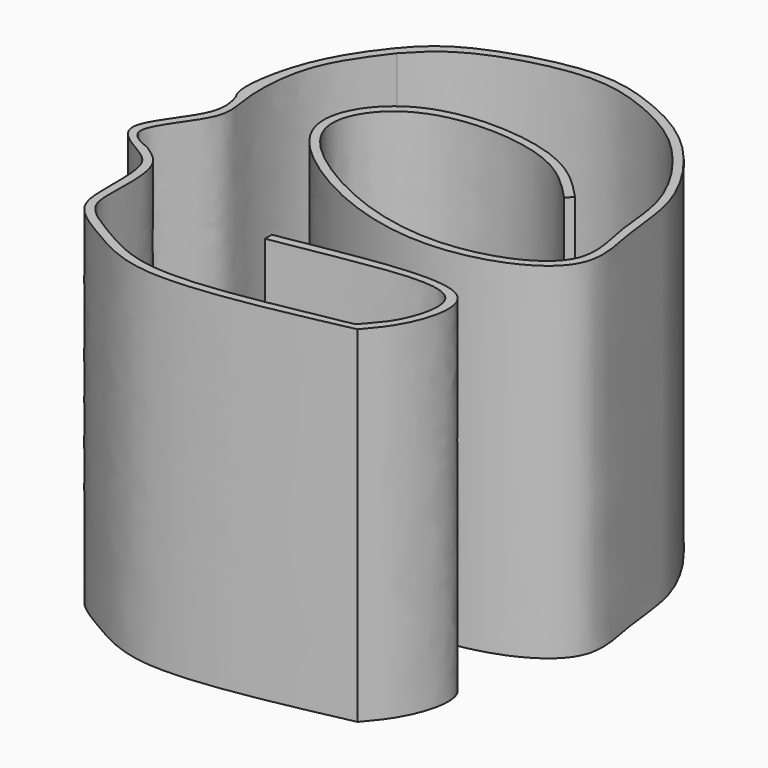
from build123d import *

# Parameters (mm, degrees)
F1_DEPTH = 50.8


with BuildPart() as f1:
    # F0 (on Top) → F1 (new body)
    with BuildSketch(Plane.XY):
        with BuildLine():
            add(Edge.make_bspline(
                [(-28.575, 9.525), (-28.8594996524, 11.5470812082), (-27.583625005, 19.7918515313), (-21.4722499031, 28.8714189263), (-15.4604819758, 34.6419109157), (0.1643363583, 39.2567574305), (9.5913489365, 36.8064392809), (19.7669349831, 31.7301076931), (28.1092618759, 19.3070522169), (28.01926673, 9.7948073112), (31.6466517803, -1.8420994785), (11.0037494052, -10.2224046216), (-9.6226479792, -1.5206953626), (-19.2672929112, 9.1233944662), (-10.4717480482, 22.0348756544), (10.3975685161, 20.7312450611), (15.7068943524, 15.1190361927), (17.9692939765, 12.7248933616)],
                knots=[0.0268047416, 0.0268047416, 0.0268047416, 0.0268047416, 0.0837333862, 0.1446640373, 0.1976117956, 0.2695895028, 0.3265181474, 0.3874487985, 0.4563906441, 0.5133192887, 0.5698365194, 0.6476379692, 0.7347556422, 0.7976731476, 0.8605906529, 0.9405180871, 1, 1, 1, 1], degree=3))
            add(Edge.make_bspline(
                [(-28.575, 9.525), (-28.3385715748, 8.9386739216), (-28.1040202058, 8.3521252843), (-27.9132703579, 7.7563821144)],
                knots=[0, 0, 0, 0, 0.0285131067, 0.0285131067, 0.0285131067, 0.0285131067], degree=3))
            add(Edge.make_bspline(
                [(-27.9132703579, 7.7563821144), (-27.457568198, 6.3331492672), (-26.8867535963, 2.2383154089), (-35.3909456885, -5.8010055969), (-28.3306633549, -9.5477989192), (-25.290962526, -11.7290065998), (-25.4629784715, -19.1717840144), (-25.2886215487, -24.9312265481), (-18.5973573035, -28.8101607796), (-9.0674060529, -34.5949711254), (8.2183413475, -30.8940706711), (19.05, -28.575)],
                knots=[0.0285131067, 0.0285131067, 0.0285131067, 0.0285131067, 0.0966310342, 0.2175283955, 0.3078022388, 0.3811674198, 0.4822582987, 0.5717569993, 0.6716096703, 0.7942539425, 1, 1, 1, 1], degree=3))
            add(Edge.make_bspline(
                [(19.05, -28.575), (20.449393147, -26.9335917203), (23.340812467, -23.5739270293), (26.0434304421, -10.5220498003), (8.2297129353, -14.3884085752), (-3.314917673, -16.3747909325)],
                knots=[0, 0, 0, 0, 0.2484947009, 0.5131438955, 1, 1, 1, 1], degree=3))
            Line((-3.314917673, -16.3747909325), (-3.314917673, -17.6447909325))
            add(Edge.make_bspline(
                [(-3.314917673, -17.6447909325), (0.1127708121, -17.0365832342), (7.2444590959, -15.7711392667), (24.4759204402, -13.0813986392), (21.9819222972, -23.2539656867), (19.4703820637, -26.1495666985), (18.4845582884, -27.288039337), (18.0801026493, -27.7551224914)],
                knots=[0, 0, 0, 0, 0.2600583017, 0.5410803086, 0.7403838213, 0.8934868177, 1, 1, 1, 1], degree=3))
            add(Edge.make_bspline(
                [(18.0801026493, -27.7551224914), (15.0345243093, -28.3437785038), (8.0398635799, -29.6957217585), (-9.585799738, -32.6564215448), (-18.0642196498, -27.6964687931), (-24.2633978347, -24.0122788001), (-24.1291593864, -19.1004975599), (-23.9516284245, -11.0740502335), (-26.7089648656, -9.2408462263), (-27.8925829323, -8.4539225305)],
                knots=[0, 0, 0, 0, 0.1608506796, 0.3694194686, 0.5259568215, 0.6514567009, 0.7585607213, 0.8963594402, 1, 1, 1, 1], degree=3))
            add(Edge.make_bspline(
                [(-27.8925829323, -8.4539225305), (-29.5438355642, -7.7290194845), (-33.5867954962, -5.9541523849), (-25.2963448806, 2.6015927727), (-27.162405802, 8.0991997717), (-26.7796800648, 19.1637843035), (-22.4645149675, 24.9082864328), (-20.2827948032, 27.8126703548)],
                knots=[0, 0, 0, 0, 0.1493716357, 0.365724497, 0.5360616686, 0.7654357157, 1, 1, 1, 1], degree=3))
            add(Edge.make_bspline(
                [(-20.2827948032, 27.8126703548), (-18.6534822427, 29.5528745857), (-14.7825375405, 33.6872773464), (0.1596409555, 37.8817329306), (9.0506352198, 35.6451933741), (18.9034559835, 30.7799498212), (26.9755324876, 18.6681192726), (26.7192855021, 9.8016253637), (30.3827219691, -1.2078222302), (10.9970588246, -8.6943882218), (-8.6689055778, -0.4891080049), (-17.761138526, 9.1459809357), (-9.7895282246, 20.5115764549), (9.6041710088, 19.7455600414), (14.8637592867, 14.1761389432), (17.1532958212, 11.7517299578)],
                knots=[0, 0, 0, 0, 0.0616698181, 0.1465160593, 0.2130625953, 0.2851516815, 0.3669424489, 0.433147703, 0.4991418759, 0.5892944238, 0.6920232222, 0.7644671824, 0.8355915351, 0.928431815, 1, 1, 1, 1], degree=3))
            Line((17.1532958212, 11.7517299578), (17.9692939765, 12.7248933616))
        make_face()
        with BuildLine():
            add(Edge.make_bspline(
                [(-28.575, 9.525), (-28.3385715748, 8.9386739216), (-28.1040202058, 8.3521252843), (-27.9132703579, 7.7563821144)],
                knots=[0, 0, 0, 0, 0.0285131067, 0.0285131067, 0.0285131067, 0.0285131067], degree=3))
            add(Edge.make_bspline(
                [(-27.9132703579, 7.7563821144), (-28.1968626586, 8.2087644493), (-28.4597901387, 8.7061459399), (-28.575, 9.525)],
                knots=[0.0037511414, 0.0037511414, 0.0037511414, 0.0037511414, 0.0268047416, 0.0268047416, 0.0268047416, 0.0268047416], degree=3))
        make_face()
    extrude(amount=F1_DEPTH)


solid = f1.part
